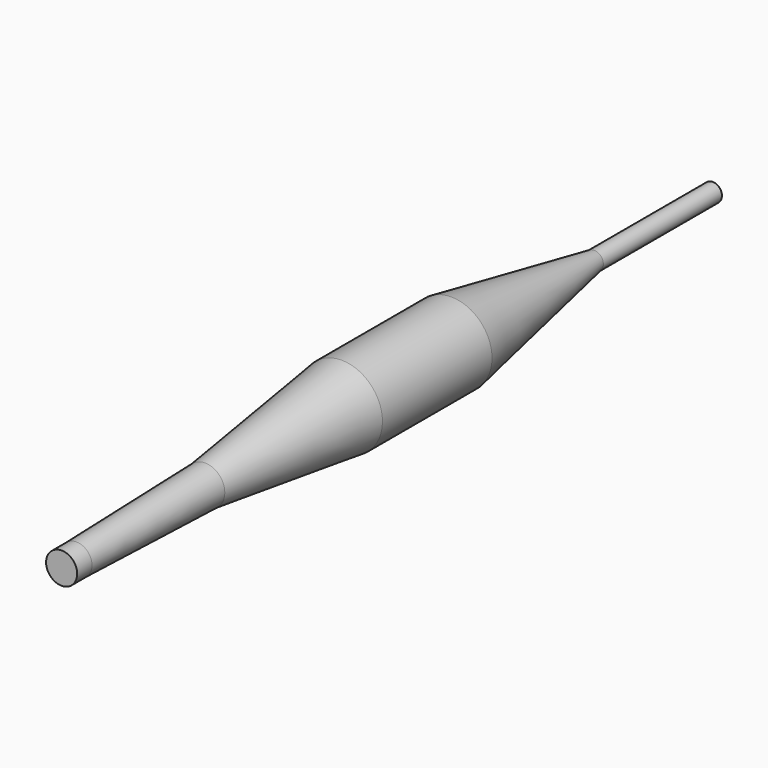
from build123d import *

# Parameters (mm, degrees)
F0_W   = 25
F0_H   = 21
F0_W_2 = 184.9109574539
F0_H_2 = 55
F0_W_3 = 200
F0_H_3 = 12.5


# Not quite as in the source:
# - the program builds the solid bodies; features that only make, move or delete a surface that nothing else refers to are left out


with BuildPart() as f1:
    # F0 (on Right) → F1 (revolve)
    with BuildSketch(Plane.YZ):
        with Locations((12.5, 223.4762815751)):
            Rectangle(F0_W, F0_H)
        Polygon((25, 233.9762815751), (25, 212.9762815751), (242, 212.9762815751), (242, 239.6586265556), align=None)
        Polygon((242, 239.6586265556), (242, 212.9762815751), (344.0616714118, 212.9762815751), (344.0616714118, 252.1902240649), align=None)
        Polygon((344.0616714118, 252.1902240649), (344.0616714118, 212.9762815751), (472.6287925066, 212.9762815751), (472.6287925066, 267.9762815751), align=None)
        with Locations((565.0842712335, 240.4762815751)):
            Rectangle(F0_W_2, F0_H_2)
        Polygon((657.5397499605, 267.9762815751), (657.5397499605, 212.9762815751), (813.5, 212.9762815751), (813.5, 240.4762815751), align=None)
        Polygon((813.5, 240.4762815751), (813.5, 212.9762815751), (898.5692272943, 212.9762815751), (898.5692272943, 225.4762815751), align=None)
        with Locations((998.5692272943, 219.2262815751)):
            Rectangle(F0_W_3, F0_H_3)
    revolve(axis=Axis((0, -32.5, 212.9762815751), (0, -1, 0)))


solid = f1.part
